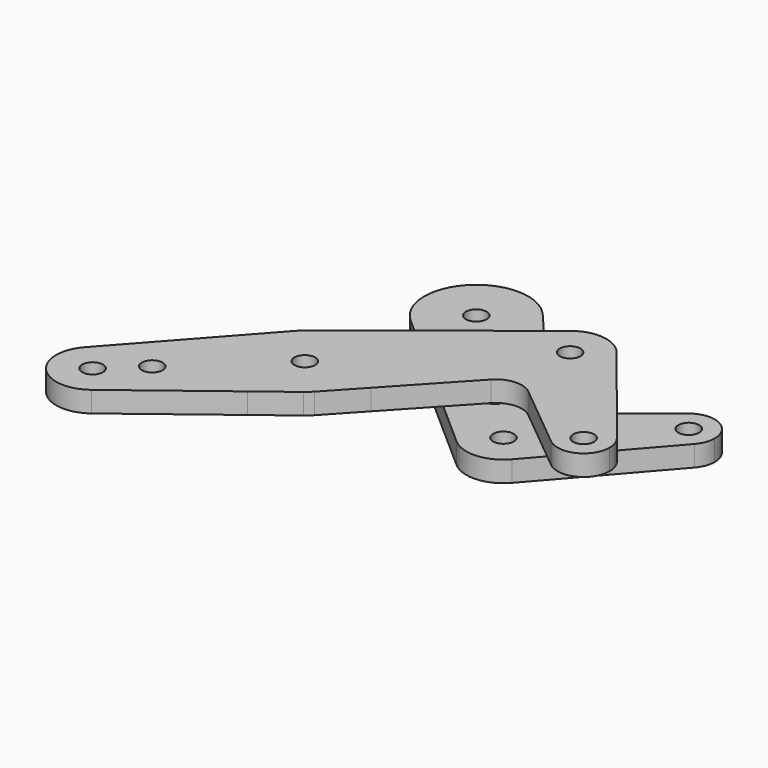
from build123d import *

# Parameters (mm, degrees)
F0_R     = 0.125
F1_DEPTH = 0.25
F2_R     = 0.125
F3_DEPTH = 0.25


# Not quite as in the source:
# - ends of sketch curves that miss each other by under 0.0002 mm in the source are joined


with BuildPart() as f1:
    # F0 (on Top) → F1 (new body)
    with BuildSketch(Plane.XY):
        with BuildLine():
            Line((-2.2996791372, -1.2826026726), (-3.6269232135, -2.7669432373))
            ThreePointArc((-3.6269232135, -2.7669432373), (-3.3095959941, -2.6211509221), (-2.9866564556, -2.7540494466))
            ThreePointArc((-2.9866564556, -2.7540494466), (-2.929558128, -2.5584979333), (-2.7635556745, -2.6765817968))
            ThreePointArc((-2.7635556745, -2.6765817968), (-2.8383720153, -2.7910658584), (-2.9732612801, -2.7685054629))
            ThreePointArc((-2.9732612801, -2.7685054629), (-2.8917036664, -2.9034596896), (-2.8632873376, -3.0585622361))
            ThreePointArc((-2.8632873376, -3.0585622361), (-2.9085080639, -3.2522713516), (-3.0348220642, -3.4059362756))
            Line((-3.0348220642, -3.4059362756), (-1.8725849919, -2.5160750152))
            Line((-1.8725849919, -2.5160750152), (-2.2590622172, -2.1571883185))
            ThreePointArc((-2.2590622172, -2.1571883185), (-2.4580978323, -1.7281958222), (-2.2996791372, -1.2826026726))
        make_face()
        with BuildLine():
            ThreePointArc((-2.9866564556, -2.7540494466), (-3.3095959941, -2.6211509221), (-3.6269232135, -2.7669432373))
            ThreePointArc((-3.6269232135, -2.7669432373), (-3.6216972176, -3.3559224535), (-3.0348220642, -3.4059362756))
            ThreePointArc((-3.0348220642, -3.4059362756), (-2.9085080639, -3.2522713516), (-2.8632873376, -3.0585622361))
            ThreePointArc((-2.8632873376, -3.0585622361), (-2.8917036664, -2.9034596896), (-2.9732612801, -2.7685054629))
            ThreePointArc((-2.9732612801, -2.7685054629), (-2.9802442117, -2.7615418589), (-2.9866564556, -2.7540494466))
        make_face()
        with Locations((-3.3007873376, -3.0585622361)):
            Circle(F0_R, mode=Mode.SUBTRACT)
        with BuildLine():
            Line((-0.2724544714, 0.3423080645), (-2.2229914165, -1.2101897215))
            ThreePointArc((-2.2229914165, -1.2101897215), (-1.7632079583, -1.0781973023), (-1.3447592224, -1.3099805689))
            Line((-1.3447592224, -1.3099805689), (-1.0099910743, -1.7305786829))
            Line((-1.0099910743, -1.7305786829), (-0.235769164, -0.8968360602))
            ThreePointArc((-0.235769164, -0.8968360602), (-0.0159442132, -0.796967297), (0.2095545573, -0.8832637821))
            Line((0.2095545573, -0.8832637821), (0.9911066788, -1.5251344451))
            ThreePointArc((0.9911066788, -1.5251344451), (0.967333205, -1.0638113252), (1.4288770162, -1.0828247256))
            Line((1.4288770162, -1.0828247256), (0.3413302011, 0.2736785411))
            ThreePointArc((0.3413302011, 0.2736785411), (0.4127579272, 0.1450418682), (0.4375, 0))
            ThreePointArc((0.4375, 0), (-0.1900097613, -0.3940844334), (-0.2724544714, 0.3423080645))
        make_face()
        with BuildLine():
            Line((-1.0099910743, -1.7305786829), (-1.3447592224, -1.3099805689))
            ThreePointArc((-1.3447592224, -1.3099805689), (-1.2437465061, -1.493054693), (-1.2087707431, -1.6992012423))
            ThreePointArc((-1.2087707431, -1.6992012423), (-1.2520204003, -1.9276559176), (-1.3757836668, -2.1244927164))
            Line((-1.3757836668, -2.1244927164), (-1.0099910743, -1.7305786829))
        make_face()
        with BuildLine():
            Line((-2.2590622172, -2.1571883185), (-1.8725849919, -2.5160750152))
            Line((-1.8725849919, -2.5160750152), (-1.4538203525, -2.1954498702))
            ThreePointArc((-1.4538203525, -2.1954498702), (-1.8634345266, -2.3234968933), (-2.2590622172, -2.1571883185))
        make_face()
        with BuildLine():
            ThreePointArc((1.5019408696, -1.2836395202), (1.4831073861, -1.1767927743), (1.4288770162, -1.0828247256))
            ThreePointArc((1.4288770162, -1.0828247256), (0.967333205, -1.0638113252), (0.9911066788, -1.5251344451))
            ThreePointArc((0.9911066788, -1.5251344451), (1.3230013716, -1.5661600368), (1.5019408696, -1.2836395202))
        make_face()
        with Locations((1.1894408696, -1.2836395202)):
            Circle(F0_R, mode=Mode.SUBTRACT)
        with BuildLine():
            ThreePointArc((0.3413302011, 0.2736785411), (0.0486155264, 0.434790502), (-0.2724544714, 0.3423080645))
            ThreePointArc((-0.2724544714, 0.3423080645), (-0.1900097613, -0.3940844334), (0.4375, 0))
            ThreePointArc((0.4375, 0), (0.4127579272, 0.1450418682), (0.3413302011, 0.2736785411))
        make_face()
        Circle(F0_R, mode=Mode.SUBTRACT)
        with BuildLine():
            ThreePointArc((-2.2229914165, -1.2101897215), (-2.2628655338, -1.2447756041), (-2.2996791372, -1.2826026726))
            ThreePointArc((-2.2996791372, -1.2826026726), (-2.4580978323, -1.7281958222), (-2.2590622172, -2.1571883185))
            ThreePointArc((-2.2590622172, -2.1571883185), (-1.8634345266, -2.3234968933), (-1.4538203525, -2.1954498702))
            ThreePointArc((-1.4538203525, -2.1954498702), (-1.4133025172, -2.161620393), (-1.3757836668, -2.1244927164))
            ThreePointArc((-1.3757836668, -2.1244927164), (-1.2520204003, -1.9276559176), (-1.2087707431, -1.6992012423))
            ThreePointArc((-1.2087707431, -1.6992012423), (-1.2437465061, -1.493054693), (-1.3447592224, -1.3099805689))
            ThreePointArc((-1.3447592224, -1.3099805689), (-1.7632079583, -1.0781973023), (-2.2229914165, -1.2101897215))
        make_face()
        with Locations((-1.8337707431, -1.6992012423)):
            Circle(F0_R, mode=Mode.SUBTRACT)
    extrude(amount=F1_DEPTH)


with BuildPart() as f3:
    # F2 (on Top) → F3 (new body)
    with BuildSketch(Plane.XY):
        with BuildLine():
            ThreePointArc((-1.870700672, -0.0590971542), (-1.200201281, -0.1598547273), (-0.8324240634, 0.4097604412))
            ThreePointArc((-0.8324240634, 0.4097604412), (-0.8710081498, 0.6259579813), (-0.9819964676, 0.8154618107))
            ThreePointArc((-0.9819964676, 0.8154618107), (-1.8958063533, 0.8552331878), (-1.870700672, -0.0590971542))
        make_face()
        with Locations((-1.4574240634, 0.4097604412)):
            Circle(F2_R, mode=Mode.SUBTRACT)
        with BuildLine():
            ThreePointArc((-0.9819964676, 0.8154618107), (-0.8710081498, 0.6259579813), (-0.8324240634, 0.4097604412))
            ThreePointArc((-0.8324240634, 0.4097604412), (-1.200201281, -0.1598547273), (-1.870700672, -0.0590971542))
            Line((-1.870700672, -0.0590971542), (0, -1.708034565))
            ThreePointArc((0, -1.708034565), (0.1117499025, -0.9643858319), (0.7435082666, -1.3722863692))
            ThreePointArc((0.7435082666, -1.3722863692), (0.7151127049, -1.529165986), (0.6335291351, -1.6661391338))
            Line((0.6335291351, -1.6661391338), (1.7790889936, -0.3501030424))
            ThreePointArc((1.7790889936, -0.3501030424), (1.3179886014, -0.3613874071), (1.3478948326, 0.0988804778))
            Line((1.3478948326, 0.0988804778), (0.5736895844, -0.5218772581))
            ThreePointArc((0.5736895844, -0.5218772581), (0.3526119109, -0.5981064496), (0.1404071565, -0.4998447095))
            Line((0.1404071565, -0.4998447095), (-0.9819964676, 0.8154618107))
        make_face()
        with Locations((-0.274249447, -0.7927647465)):
            Circle(F2_R, mode=Mode.SUBTRACT)
        with BuildLine():
            ThreePointArc((0.7435082666, -1.3722863692), (0.1117499025, -0.9643858319), (0, -1.708034565))
            ThreePointArc((0, -1.708034565), (0.3254795809, -1.8188724567), (0.6335291351, -1.6661391338))
            ThreePointArc((0.6335291351, -1.6661391338), (0.7151127049, -1.529165986), (0.7435082666, -1.3722863692))
        make_face()
        with Locations((0.2959467375, -1.3722863692)):
            Circle(F2_R, mode=Mode.SUBTRACT)
        with BuildLine():
            ThreePointArc((1.8558795048, -0.1449268086), (1.6785965339, 0.1368046327), (1.3478948326, 0.0988804778))
            ThreePointArc((1.3478948326, 0.0988804778), (1.3179886014, -0.3613874071), (1.7790889936, -0.3501030424))
            ThreePointArc((1.7790889936, -0.3501030424), (1.8360529279, -0.2544645527), (1.8558795048, -0.1449268086))
        make_face()
        with Locations((1.5433795048, -0.1449268086)):
            Circle(F2_R, mode=Mode.SUBTRACT)
    extrude(amount=-F3_DEPTH)


solid = Compound([f1.part, f3.part])
